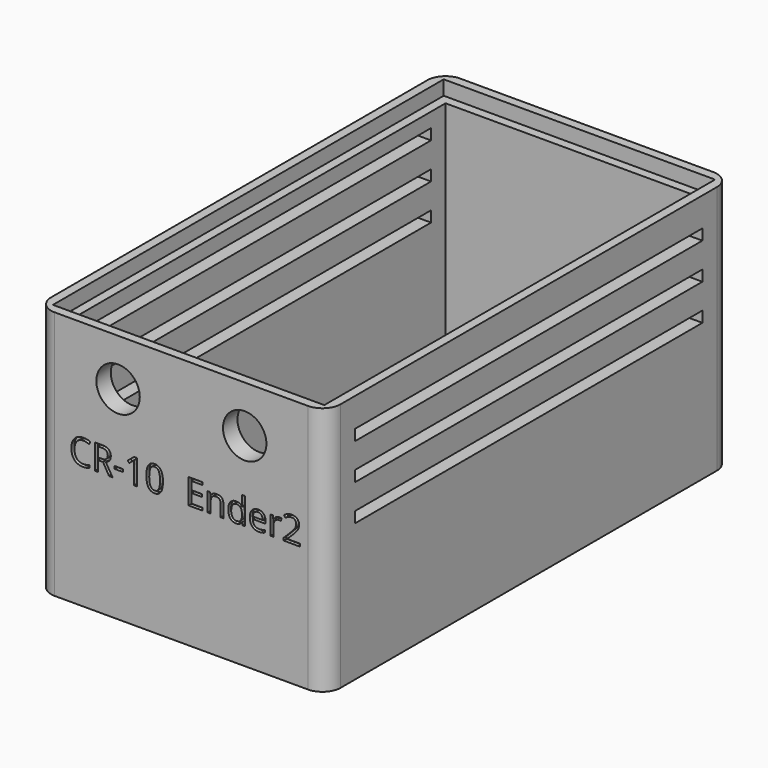
from build123d import *

# Parameters (mm, degrees)
F0_W          = 80
F0_H          = 140
F1_DEPTH      = 4
F2_W          = 80
F2_H          = 140
F2_W_2        = 70
F2_H_2        = 130
F3_DEPTH      = 65
F4_R          = 5
F5_DEPTH      = 25
F6_W          = 120
F6_H          = 3
F7_DEPTH      = 100
F8_R          = 5
F9_W          = 75
F9_H          = 135
F9_W_2        = 70
F9_H_2        = 130
F10_DEPTH     = 4
F11_R         = 6
F12_DEPTH     = 25
F11_TEXT_SIZE = 9.7222222222
F13_DEPTH     = 1


# Not quite as in the source:
# - Text() gives the source's letters only with a copy of the font that has no kerning and outlines rounded to 1/6400 em; it was checked with that copy


with BuildPart() as f1:
    # F0 (on Top) → F1 (new body)
    with BuildSketch(Plane.XY):
        Rectangle(F0_W, F0_H)
    extrude(amount=F1_DEPTH)

    # F2 (on face) → F3 (join)
    with BuildSketch(Plane.XY.offset(4)):
        Rectangle(F2_W, F2_H)
        Rectangle(F2_W_2, F2_H_2, mode=Mode.SUBTRACT)
    extrude(amount=F3_DEPTH)

    # F4 (on face) → F5 (cut)
    with BuildSketch(Plane(origin=(0, 70, 0), x_dir=(-1, 0, 0), z_dir=(0, 1, 0))):
        with Locations((-20, 10)):
            Circle(F4_R)
        with Locations((0, 10)):
            Circle(F4_R)
        with Locations((20, 10)):
            Circle(F4_R)
    extrude(amount=-F5_DEPTH, mode=Mode.SUBTRACT)

    # F6 (on face) → F7 (cut)
    with BuildSketch(Plane.YZ.offset(40)):
        with Locations((0, 59.5)):
            Rectangle(F6_W, F6_H)
        with Locations((0, 49.5)):
            Rectangle(F6_W, F6_H)
        with Locations((0, 39.5)):
            Rectangle(F6_W, F6_H)
    extrude(amount=-F7_DEPTH, mode=Mode.SUBTRACT)

    # F8
    f8_edges = [f1.edges().sort_by_distance(p)[0] for p in [
        (-40, -70, 34.5),
        (40, -70, 34.5),
        (-40, 70, 34.5),
        (40, 70, 34.5),
    ]]
    fillet(f8_edges, radius=F8_R)

    # F9 (on face) → F10 (cut)
    with BuildSketch(Plane.XY.offset(69)):
        Rectangle(F9_W, F9_H)
        Rectangle(F9_W_2, F9_H_2, mode=Mode.SUBTRACT)
    extrude(amount=-F10_DEPTH, mode=Mode.SUBTRACT)

    # F11 (on face) → F12 (cut)
    with BuildSketch(Plane.XZ.offset(70)):
        with Locations((-17.5, 56.0454410116)):
            Circle(F11_R)
        with Locations((17.5, 56.0454410116)):
            Circle(F11_R)
    extrude(amount=-F12_DEPTH, mode=Mode.SUBTRACT)

    # F11 (on face) → F13 (cut)
    with BuildSketch(Plane.XZ.offset(70)):
        with Locations((-17.5, 56.0454410116)):
            Circle(F11_R)
        with Locations((17.5, 56.0454410116)):
            Circle(F11_R)
        with Locations((-31, 34.0454410116)):
            Text('CR-10', F11_TEXT_SIZE, font='Open Sans', text_align=(TextAlign.LEFT, TextAlign.BOTTOM))
        with Locations((1.0355902778, 34.0454410116)):
            Text('Ender2', F11_TEXT_SIZE, font='Open Sans', text_align=(TextAlign.LEFT, TextAlign.BOTTOM))
    extrude(amount=-F13_DEPTH, mode=Mode.SUBTRACT)


solid = f1.part
